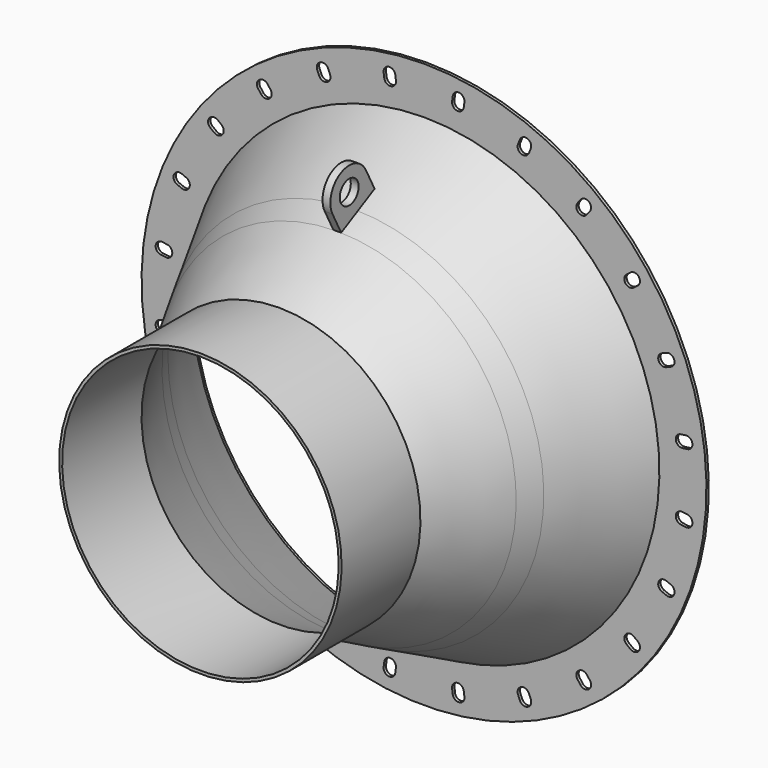
from build123d import *

# Parameters (mm, degrees)
F3_W            = 4.7625
F3_H            = 76.2
F6_T            = -4.7625
F8_DEPTH        = 4.7625
F8_COPIES_COUNT = 24
F3_R            = 19.05
F9_DEPTH        = 6.35


# Not quite as in the source:
# - a pattern or mirror of a feature is missing from the dataset's text; its kind, count and spacing are read off the source's solid


with BuildPart() as f4:
    # F3 (on Right) → F4 (revolve)
    with BuildSketch(Plane.YZ):
        with Locations((-2.38125, 419.1)):
            Rectangle(F3_W, F3_H)
    revolve(axis=Axis((0, -209.601546452, 0), (0, -1, 0)))

    # F7 (on Front) → F8 (cut, through all)
    with BuildSketch(Plane.XZ):
        with BuildLine():
            Line((64.3542497942, 415.8451981383), (65.3903014449, 423.7147917255))
            ThreePointArc((65.3903014449, 423.7147917255), (57.1836583904, 434.3530083993), (46.5032768357, 426.2013156872))
            Line((46.5032768357, 426.2013156872), (45.467225185, 418.3317221001))
            ThreePointArc((45.467225185, 418.3317221001), (53.6582850209, 407.5751391295), (64.3542497942, 415.8451981383))
        make_face()
    f8 = extrude(amount=F8_DEPTH, mode=Mode.SUBTRACT)

    # F8_copies: F8 ×24 about axis
    f8_copies_axis = Axis((0, 0, 0), (0, 1, 0))
    for i in range(1, F8_COPIES_COUNT):
        add(f8.rotate(f8_copies_axis, i * 360 / F8_COPIES_COUNT), mode=Mode.SUBTRACT)


with BuildPart() as f5:
    # F3 (on Right) → F5 (revolve)
    with BuildSketch(Plane.YZ):
        Polygon((0, 381), (-4.7625, 381), (-112.674705011, 324.856950721), (-146.4739859916, 307.2723346204), (-180.2732642198, 289.6877199517), (-297.6895899046, 228.6), (-457.2, 228.6), (-457.2, 0), (0, 0), align=None)
    revolve(axis=Axis((0, -209.601546452, 0), (0, -1, 0)))

    # F6
    f6_openings = [f5.faces().sort_by_distance(p)[0] for p in [
        (0, -457.2, 0),
        (0, 0, 0),
    ]]
    offset(amount=F6_T, openings=f6_openings, kind=Kind.INTERSECTION)


with BuildPart() as f9:
    # F3 (on Right) → F9 (new body, symmetric)
    with BuildSketch(Plane.YZ):
        with BuildLine():
            ThreePointArc((-197.8578796044, 323.4869995561), (-175.5240997642, 304.7377145837), (-146.4739859916, 307.2723346204))
            ThreePointArc((-146.4739859916, 307.2723346204), (-131.488799619, 321.3024950023), (-125.9586, 341.0716149407))
            ThreePointArc((-125.9586, 341.0716149407), (-127.0493947064, 350.123063639), (-130.2593203956, 358.6562303254))
            ThreePointArc((-130.2593203956, 358.6562303254), (-181.6432153846, 374.8708945451), (-197.8578796044, 323.4869995561))
        make_face()
        with Locations((-164.0586, 341.0716149407)):
            Circle(F3_R, mode=Mode.SUBTRACT)
        with BuildLine():
            Line((-180.2732642198, 289.6877199517), (-146.4739859916, 307.2723346204))
            ThreePointArc((-146.4739859916, 307.2723346204), (-175.5240997642, 304.7377145837), (-197.8578796044, 323.4869995561))
            Line((-197.8578796044, 323.4869995561), (-180.2732642198, 289.6877199517))
        make_face()
        with BuildLine():
            Line((-146.4739859916, 307.2723346204), (-112.674705011, 324.856950721))
            Line((-112.674705011, 324.856950721), (-130.2593203956, 358.6562303254))
            ThreePointArc((-130.2593203956, 358.6562303254), (-127.0493947064, 350.123063639), (-125.9586, 341.0716149407))
            ThreePointArc((-125.9586, 341.0716149407), (-131.488799619, 321.3024950023), (-146.4739859916, 307.2723346204))
        make_face()
    extrude(amount=F9_DEPTH, both=True)


solid = Compound([f4.part, f5.part, f9.part])
